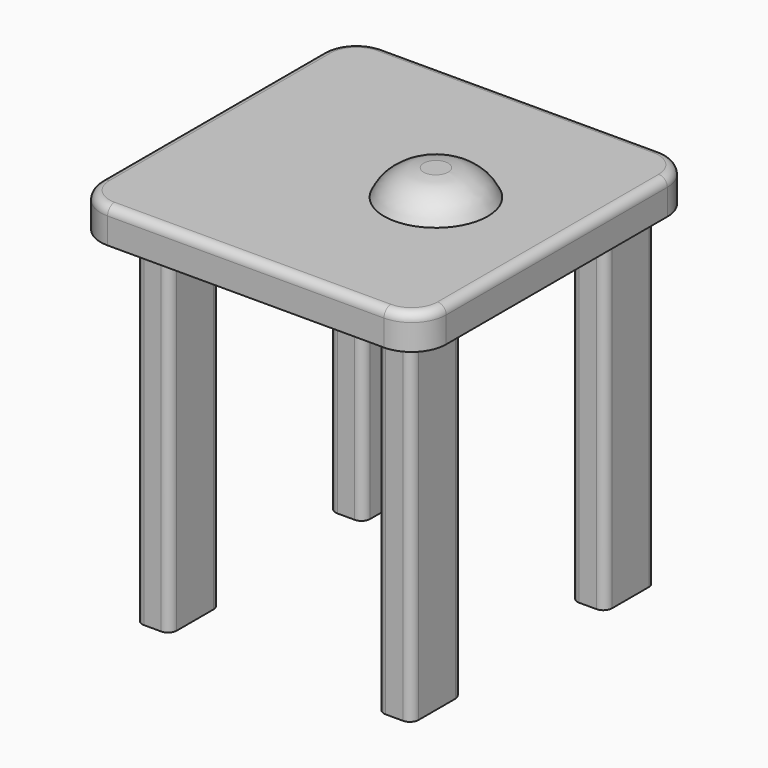
from build123d import *

# Parameters (mm, degrees)
F1_DEPTH = 40
F2_R     = 10
F4_DEPTH = 400
F5_R     = 60.0444611856
F6_DEPTH = 30


# Not quite as in the source:
# - a fillet or chamfer that OpenCascade refuses, or shapes differently, is made with other operations: its cross-section is extruded or revolved along the edge and cut away or added


with BuildPart() as f1:
    # F0 (on Top) → F1 (new body)
    with BuildSketch(Plane.XY):
        with BuildLine():
            ThreePointArc((-260.7041027397, -159.2581299295), (-248.9883739872, -187.542401177), (-220.7041027397, -199.2581299295))
            Line((-220.7041027397, -199.2581299295), (99.2958972603, -199.2581299295))
            ThreePointArc((99.2958972603, -199.2581299295), (127.5801685078, -187.542401177), (139.2958972603, -159.2581299295))
            Line((139.2958972603, -159.2581299295), (139.2958972603, 160.7418700705))
            ThreePointArc((139.2958972603, 160.7418700705), (127.5801685078, 189.0261413179), (99.2958972603, 200.7418700705))
            Line((99.2958972603, 200.7418700705), (-220.7041027397, 200.7418700705))
            ThreePointArc((-220.7041027397, 200.7418700705), (-248.9883739872, 189.0261413179), (-260.7041027397, 160.7418700705))
            Line((-260.7041027397, 160.7418700705), (-260.7041027397, -159.2581299295))
        make_face()
    extrude(amount=F1_DEPTH)

    # F2
    f2_edges = [f1.edges().sort_by_distance(p)[0] for p in [
        (-260.704103, 0.74187, 40),
        (-248.988374, -187.542401, 40),
        (-60.704103, -199.25813, 40),
        (127.580169, -187.542401, 40),
        (139.295897, 0.74187, 40),
        (127.580169, 189.026141, 40),
        (-60.704103, 200.74187, 40),
        (-248.988374, 189.026141, 40),
    ]]
    fillet(f2_edges, radius=F2_R)

    # F3 (on face) → F4 (join)
    with BuildSketch(Plane(origin=(0, 0, 0), x_dir=(1, 0, 0), z_dir=(0, 0, -1))):
        with BuildLine():
            Line((99.2958972603, -184.0014514797), (99.2958972603, -130.7418700705))
            ThreePointArc((99.2958972603, -130.7418700705), (96.3669650722, -123.6708022586), (89.2958972603, -120.7418700705))
            Line((89.2958972603, -120.7418700705), (69.2958972603, -120.7418700705))
            ThreePointArc((69.2958972603, -120.7418700705), (62.2248294484, -123.6708022586), (59.2958972603, -130.7418700705))
            Line((59.2958972603, -130.7418700705), (59.2958972603, -184.0014514797))
            ThreePointArc((59.2958972603, -184.0014514797), (62.2248294484, -191.0725192915), (69.2958972603, -194.0014514797))
            Line((69.2958972603, -194.0014514797), (89.2958972603, -194.0014514797))
            ThreePointArc((89.2958972603, -194.0014514797), (96.3669650722, -191.0725192915), (99.2958972603, -184.0014514797))
        make_face()
        with BuildLine():
            ThreePointArc((99.2958972603, 149.2581299295), (96.3669650722, 156.3291977414), (89.2958972603, 159.2581299295))
            Line((89.2958972603, 159.2581299295), (69.2958972603, 159.2581299295))
            ThreePointArc((69.2958972603, 159.2581299295), (62.2248294484, 156.3291977414), (59.2958972603, 149.2581299295))
            Line((59.2958972603, 149.2581299295), (59.2958972603, 95.9985485203))
            ThreePointArc((59.2958972603, 95.9985485203), (62.2248294484, 88.9274807085), (69.2958972603, 85.9985485203))
            Line((69.2958972603, 85.9985485203), (89.2958972603, 85.9985485203))
            ThreePointArc((89.2958972603, 85.9985485203), (96.3669650722, 88.9274807085), (99.2958972603, 95.9985485203))
            Line((99.2958972603, 95.9985485203), (99.2958972603, 149.2581299295))
        make_face()
        with BuildLine():
            Line((-180.7041027397, 95.9985485203), (-180.7041027397, 149.2581299295))
            ThreePointArc((-180.7041027397, 149.2581299295), (-183.6330349278, 156.3291977414), (-190.7041027397, 159.2581299295))
            Line((-190.7041027397, 159.2581299295), (-210.7041027397, 159.2581299295))
            ThreePointArc((-210.7041027397, 159.2581299295), (-217.7751705516, 156.3291977414), (-220.7041027397, 149.2581299295))
            Line((-220.7041027397, 149.2581299295), (-220.7041027397, 95.9985485203))
            ThreePointArc((-220.7041027397, 95.9985485203), (-217.7751705516, 88.9274807085), (-210.7041027397, 85.9985485203))
            Line((-210.7041027397, 85.9985485203), (-190.7041027397, 85.9985485203))
            ThreePointArc((-190.7041027397, 85.9985485203), (-183.6330349278, 88.9274807085), (-180.7041027397, 95.9985485203))
        make_face()
        with BuildLine():
            Line((-180.7041027397, -184.0014514797), (-180.7041027397, -130.7418700705))
            ThreePointArc((-180.7041027397, -130.7418700705), (-183.6330349278, -123.6708022586), (-190.7041027397, -120.7418700705))
            Line((-190.7041027397, -120.7418700705), (-210.7041027397, -120.7418700705))
            ThreePointArc((-210.7041027397, -120.7418700705), (-217.7751705516, -123.6708022586), (-220.7041027397, -130.7418700705))
            Line((-220.7041027397, -130.7418700705), (-220.7041027397, -184.0014514797))
            ThreePointArc((-220.7041027397, -184.0014514797), (-217.7751705516, -191.0725192915), (-210.7041027397, -194.0014514797))
            Line((-210.7041027397, -194.0014514797), (-190.7041027397, -194.0014514797))
            ThreePointArc((-190.7041027397, -194.0014514797), (-183.6330349278, -191.0725192915), (-180.7041027397, -184.0014514797))
        make_face()
    extrude(amount=F4_DEPTH)

    # F5 (on face) → F6 (join)
    with BuildSketch(Plane.XY.offset(40)):
        Circle(F5_R)
    extrude(amount=F6_DEPTH)

    # F7: fillet of radius 50 on 1 edges, made by hand

    # F7_s1 → F7_t2 (revolve, cut)
    with BuildSketch(Plane.XZ):
        with BuildLine():
            ThreePointArc((60.0444611856, 40), (41.6048321113, 61.8330013267), (14.218704236, 70))
            Line((14.218704236, 70), (60.0444611856, 70))
            Line((60.0444611856, 70), (60.0444611856, 40))
        make_face()
    revolve(axis=Axis((0, 0, 70), (0, 0, 1)), mode=Mode.SUBTRACT)


solid = f1.part
